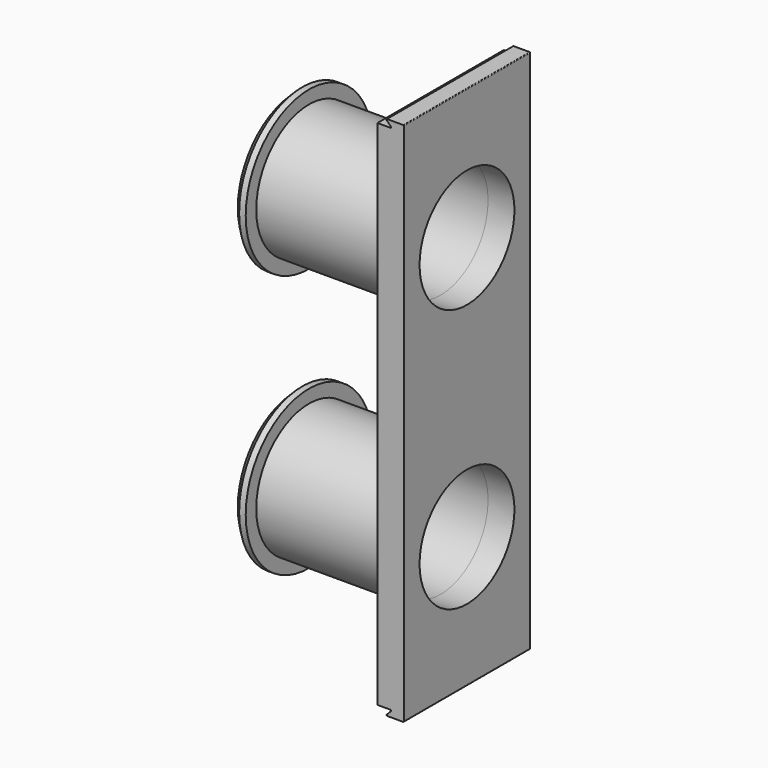
from build123d import *

# Parameters (mm, degrees)
F1_DEPTH = 12
F2_R     = 5
F2_R_2   = 4.5
F3_DEPTH = 10
F4_R     = 6
F4_R_2   = 4.5
F5_DEPTH = 1
F6_DEPTH = 25
F7_SIZE  = 0.5


with BuildPart() as f1:
    # F0 (on Front) → F1 (new body)
    with BuildSketch(Plane.XZ):
        with BuildLine():
            Line((-5.8526312746, -17.3661426386), (-5.8526312746, 22.4338573614))
            ThreePointArc((-5.8526312746, 22.4338573614), (-5.8672759356, 22.4692127005), (-5.9026312746, 22.4838573614))
            Line((-5.9026312746, 22.4838573614), (-7.1112099184, 22.4838573614))
            ThreePointArc((-7.1112099184, 22.4838573614), (-7.157403895, 22.452991533), (-7.1465652574, 22.3985020224))
            Line((-7.1465652574, 22.3985020224), (-6.8172759356, 22.0692127005))
            ThreePointArc((-6.8172759356, 22.0692127005), (-6.806437298, 22.0147231898), (-6.8526312746, 21.9838573614))
            Line((-6.8526312746, 21.9838573614), (-7.8526312746, 21.9838573614))
            Line((-7.8526312746, 21.9838573614), (-7.8526312746, -16.9161426386))
            Line((-7.8526312746, -16.9161426386), (-6.8526312746, -16.9161426386))
            ThreePointArc((-6.8526312746, -16.9161426386), (-6.806437298, -16.947008467), (-6.8172759356, -17.0014979776))
            Line((-6.8172759356, -17.0014979776), (-7.1465652574, -17.3307872995))
            ThreePointArc((-7.1465652574, -17.3307872995), (-7.157403895, -17.3852768102), (-7.1112099184, -17.4161426386))
            Line((-7.1112099184, -17.4161426386), (-5.9026312746, -17.4161426386))
            ThreePointArc((-5.9026312746, -17.4161426386), (-5.8672759356, -17.4014979776), (-5.8526312746, -17.3661426386))
        make_face()
    extrude(amount=F1_DEPTH)

    # F2 (on face) → F3 (join)
    with BuildSketch(Plane(origin=(-7.8526312746, 0, 0), x_dir=(0, -1, 0), z_dir=(-1, 0, 0))):
        with Locations((6, 12.5338573614)):
            Circle(F2_R)
        with Locations((6, 12.5338573614)):
            Circle(F2_R_2, mode=Mode.SUBTRACT)
        with Locations((6, -7.4661426386)):
            Circle(F2_R)
        with Locations((6, -7.4661426386)):
            Circle(F2_R_2, mode=Mode.SUBTRACT)
    extrude(amount=F3_DEPTH)

    # F4 (on face) → F5 (join)
    with BuildSketch(Plane(origin=(-17.8526312746, 0, 0), x_dir=(0, -1, 0), z_dir=(-1, 0, 0))):
        with Locations((6, 12.5338573614)):
            Circle(F4_R)
        with Locations((6, 12.5338573614)):
            Circle(F4_R_2, mode=Mode.SUBTRACT)
        with Locations((6, -7.4661426386)):
            Circle(F4_R)
        with Locations((6, -7.4661426386)):
            Circle(F4_R_2, mode=Mode.SUBTRACT)
    extrude(amount=F5_DEPTH)

    # F6 (cut): faces of the model
    f6_faces = [f1.faces().sort_by_distance(p)[0] for p in [
        (-7.8526312746, -6, 12.5338573614),
        (-7.8526312746, -6, -7.4661426386),
    ]]
    extrude(f6_faces, amount=-F6_DEPTH, mode=Mode.SUBTRACT)

    # F7
    f7_edges = [f1.edges().sort_by_distance(p)[0] for p in [
        (-18.852631, 0, 12.533857),
        (-18.852631, 0, -7.466143),
    ]]
    chamfer(f7_edges, length=F7_SIZE)


solid = f1.part
